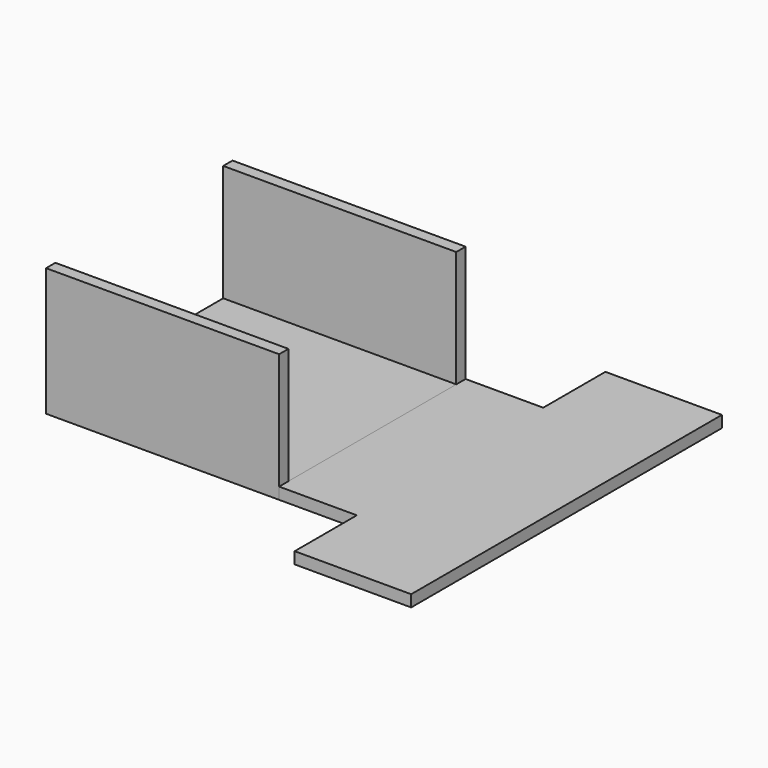
from build123d import *

# Parameters (mm, degrees)
F0_W     = 30.0000150987
F0_H     = 30
F1_DEPTH = 1.5
F3_DEPTH = 1.5
F4_W     = 30.0000150987
F4_H     = 1.5
F5_DEPTH = 15
F6_W     = 30.0000150987
F6_H     = 1.5
F7_DEPTH = 15


with BuildPart() as f1:
    # F0 (on Top) → F1 (new body)
    with BuildSketch(Plane.XY):
        Rectangle(F0_W, F0_H)
    extrude(amount=F1_DEPTH)

    # F4 (on face) → F5 (join)
    with BuildSketch(Plane.XY.offset(1.5)):
        with Locations((0, 14.25)):
            Rectangle(F4_W, F4_H)
    extrude(amount=F5_DEPTH)

    # F6 (on face) → F7 (join)
    with BuildSketch(Plane.XY.offset(1.5)):
        with Locations((0, -14.25)):
            Rectangle(F6_W, F6_H)
    extrude(amount=F7_DEPTH)


with BuildPart() as f3:
    # F2 (on face) → F3 (new body)
    with BuildSketch(Plane.XY.offset(1.5)):
        Polygon((25.0000075493, 15), (15.0000075493, 15), (15.0000075493, -15), (25.0000075493, -15), (25.0000075493, -25), (40.0000075493, -25), (40.0000075493, 25), (25.0000075493, 25), align=None)
    extrude(amount=-F3_DEPTH)


solid = Compound([f1.part, f3.part])
